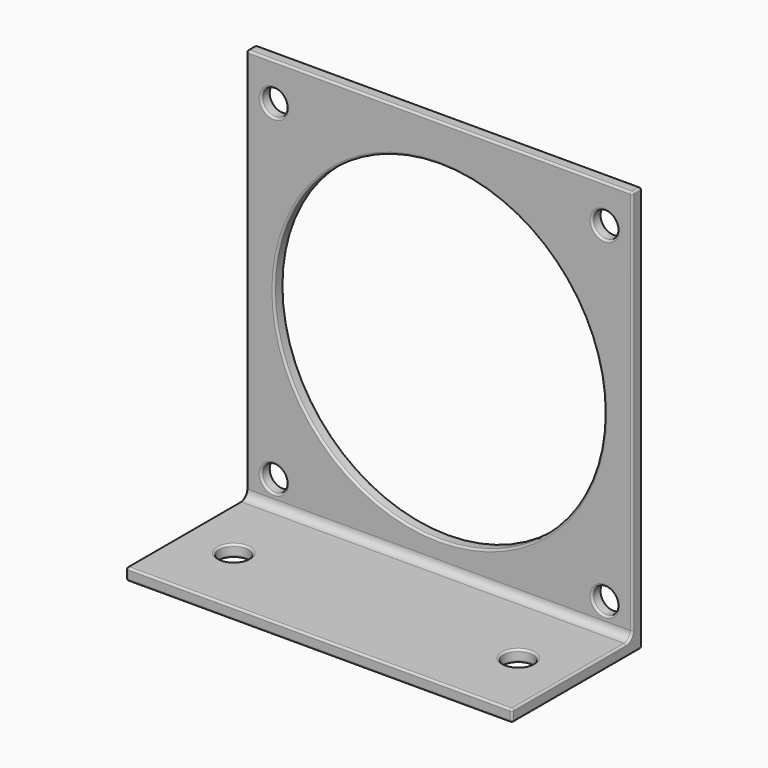
from build123d import *

# Parameters (mm, degrees)
F0_W     = 18.8
F0_H     = 1.5
F1_DEPTH = 48.3
F2_R     = 1
F4_D     = 3.18
F6_D     = 3.7
F7_D     = 41.4
F8_R     = 0.25


with BuildPart() as f1:
    # F0 (on Right) → F1 (new body)
    with BuildSketch(Plane.YZ):
        with Locations((-10.15, -24.65)):
            Rectangle(F0_W, F0_H)
        Polygon((0.75, -25.4), (0.75, 25.4), (-0.75, 25.4), (-0.75, -23.9), (-0.75, -25.4), align=None)
    extrude(amount=F1_DEPTH)

    # F2
    f2_edges = [f1.edges().sort_by_distance(p)[0] for p in [
        (24.15, -0.75, -23.9),
    ]]
    fillet(f2_edges, radius=F2_R)

    # F4 (through all)
    with Locations(Plane.XZ.offset(0.75)):
        with Locations((3.45, 20.7), (44.85, 20.7), (44.85, -20.7), (3.45, -20.7)):
            Hole(F4_D / 2)

    # F6 (through all)
    with Locations(Plane.XY.offset(-23.9)):
        with Locations((6.35, -10.65), (41.95, -10.65)):
            Hole(F6_D / 2)

    # F7 (through all)
    with Locations(Plane.XZ.offset(0.75)):
        with Locations((24.15, 0)):
            Hole(F7_D / 2)

    # F8
    f8_edges = [f1.edges().sort_by_distance(p)[0] for p in [
        (24.15, 0.75, 25.4),
        (0, 0.75, 0),
        (24.15, 0.75, -25.4),
        (48.3, 0.75, 0),
        (0, 0, 25.4),
        (48.3, 0, 25.4),
        (24.15, -0.75, 25.4),
        (48.3, -0.75, 1.25),
        (0, -0.75, 1.25),
        (0, -10.65, -23.9),
        (0, -1.042893, -23.607107),
        (48.3, -10.65, -23.9),
        (48.3, -1.042893, -23.607107),
        (0, -9.4, -25.4),
        (24.15, -19.55, -25.4),
        (0, -19.55, -24.65),
        (48.3, -9.4, -25.4),
        (24.15, -19.55, -23.9),
        (48.3, -19.55, -24.65),
        (40.1, -10.65, -23.9),
        (4.5, -10.65, -23.9),
        (40.1, -10.65, -25.4),
        (4.5, -10.65, -25.4),
        (43.26, -0.75, 20.7),
        (43.26, -0.75, -20.7),
        (1.86, -0.75, 20.7),
        (3.45, -0.75, 0),
        (1.86, -0.75, -20.7),
        (43.26, 0.75, -20.7),
        (43.26, 0.75, 20.7),
        (1.86, 0.75, -20.7),
        (3.45, 0.75, 0),
        (1.86, 0.75, 20.7),
    ]]
    fillet(f8_edges, radius=F8_R)


solid = f1.part
